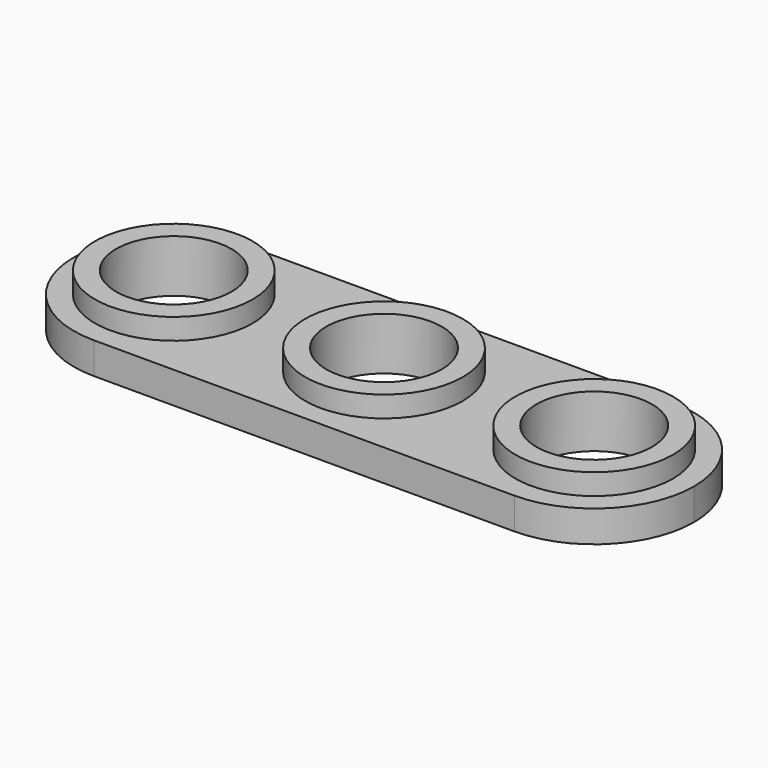
from build123d import *

# Parameters (mm, degrees)
F2_R     = 7.5
F3_DEPTH = 3
F2_R_2   = 5.5
F4_DEPTH = 5


# Not quite as in the source:
# - a feature names something its author has since deleted; it is built from what else it names


with BuildPart() as f3:
    # F2 (on Top) → F3 (new body)
    with BuildSketch(Plane.XY):
        with BuildLine():
            Line((40, 9.5), (0, 9.5))
            ThreePointArc((0, 9.5), (-6.7175144213, 6.7175144213), (-9.5, 0))
            ThreePointArc((-9.5, 0), (-6.7175144213, -6.7175144213), (0, -9.5))
            Line((0, -9.5), (40, -9.5))
            ThreePointArc((40, -9.5), (46.7175144213, -6.7175144213), (49.5, 0))
            ThreePointArc((49.5, 0), (46.7175144213, 6.7175144213), (40, 9.5))
        make_face()
        Circle(F2_R, mode=Mode.SUBTRACT)
        with Locations((20, 0)):
            Circle(F2_R, mode=Mode.SUBTRACT)
        with Locations((40, 0)):
            Circle(F2_R, mode=Mode.SUBTRACT)
    extrude(amount=F3_DEPTH)

    # F2 (on Top) → F4 (join)
    with BuildSketch(Plane.XY):
        Circle(F2_R)
        Circle(F2_R_2, mode=Mode.SUBTRACT)
        with Locations((20, 0)):
            Circle(F2_R)
        with Locations((20, 0)):
            Circle(F2_R_2, mode=Mode.SUBTRACT)
        with Locations((40, 0)):
            Circle(F2_R)
        with Locations((40, 0)):
            Circle(F2_R_2, mode=Mode.SUBTRACT)
    extrude(amount=F4_DEPTH)


solid = f3.part
